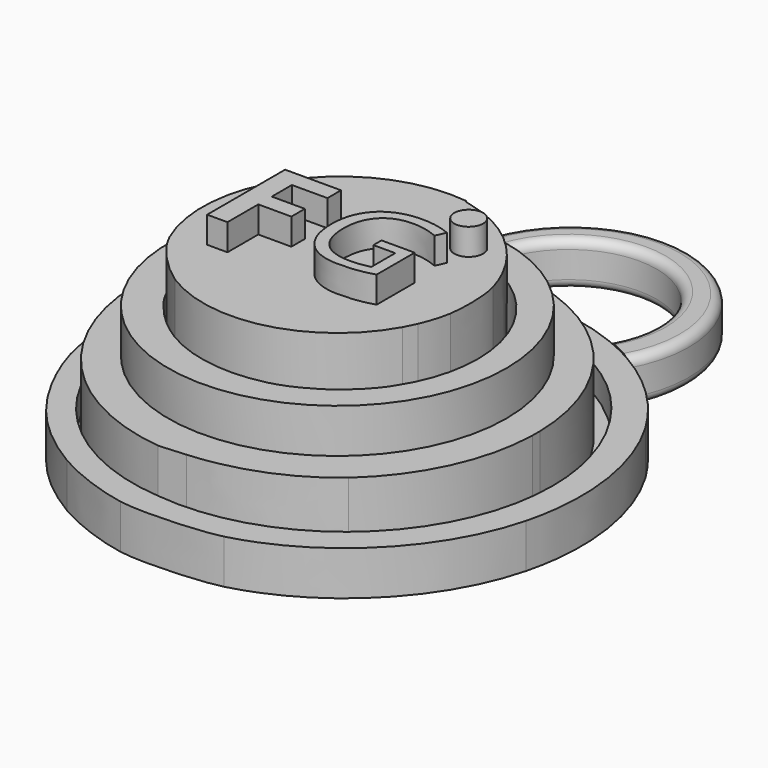
from build123d import *

# Parameters (mm, degrees)
F1_DEPTH     = 20
F0_R         = 19.1279803991
F2_DEPTH     = 15
F3_DEPTH     = 10
F4_DEPTH     = 5
F5_DEPTH     = 5
F6_R         = 1.637802748
F6_TEXT_SIZE = 15.4476677481
F7_DEPTH     = 3
F8_R         = 25.6523292118
F9_DEPTH     = 2
F10_R        = 1


# Not quite as in the source:
# - ends of sketch curves that miss each other by under 0.0002 mm in the source are joined
# - Text() gives the source's letters only with a copy of the font that has no kerning and outlines rounded to 1/6400 em; it was checked with that copy


with BuildPart() as f1:
    # F0 (on Top) → F1 (new body)
    with BuildSketch(Plane.XY):
        with BuildLine():
            ThreePointArc((-59.2347954449, -6.6814816572), (-58.8341384592, -7.4289203643), (-58.392389, -8.152832))
            add(Edge.make_bspline(
                [(-53.744252573, -12.7362436448), (-55.4325929195, -11.5891561276), (-56.9948624064, -10.0566206788), (-58.392389, -8.152832)],
                knots=[0.6895887738, 0.6895887738, 0.6895887738, 0.6895887738, 1, 1, 1, 1], degree=3))
            ThreePointArc((-53.744252573, -12.7362436448), (-41.8918676364, -14.5976951318), (-32.3863979152, -7.277170854))
            add(Edge.make_bspline(
                [(-31.7292377779, -5.9498852292), (-31.9282672637, -6.3926584279), (-32.1497491558, -6.8396976677), (-32.3863979152, -7.277170854)],
                knots=[0.3344487947, 0.3344487947, 0.3344487947, 0.3344487947, 0.5301452615, 0.5301452615, 0.5301452615, 0.5301452615], degree=3))
            ThreePointArc((-31.7292377779, -5.9498852292), (-31.1257115517, -4.3145190756), (-30.7135409768, -2.6207712256))
            add(Edge.make_bspline(
                [(-30.960104, 3.756096), (-30.5099847308, 2.24037654), (-30.4258381475, -0.5496711887), (-30.7135409768, -2.6207712256)],
                knots=[0, 0, 0, 0, 0.8296456494, 0.8296456494, 0.8296456494, 0.8296456494], degree=3))
            add(Edge.make_bspline(
                [(-42.081192, 14.696398), (-36.917409, 13.446373), (-32.566826, 9.166513), (-30.960104, 3.756096)],
                knots=[0, 0, 0, 0, 1, 1, 1, 1], degree=3))
            add(Edge.make_bspline(
                [(-43.101174, 15.090313), (-43.392217, 15.079888), (-42.933225, 14.902656), (-42.081192, 14.696398)],
                knots=[0, 0, 0, 0, 1, 1, 1, 1], degree=3))
            ThreePointArc((-43.101174, 15.090313), (-57.4988268935, 8.8957795494), (-59.2347954449, -6.6814816572))
        make_face()
    extrude(amount=F1_DEPTH)

    # F6 (on face) → F7 (join)
    with BuildSketch(Plane.XY.offset(20)):
        with Locations((-37.2399128973, 8.1431278959)):
            Circle(F6_R)
        with Locations((-57.1012012661, -5.7597728446)):
            Text('F', F6_TEXT_SIZE, font='Open Sans', font_style=FontStyle.BOLD, text_align=(TextAlign.LEFT, TextAlign.BOTTOM))
        with Locations((-46.9719469547, -5.7597728446)):
            Text('G', F6_TEXT_SIZE, font='Open Sans', text_align=(TextAlign.LEFT, TextAlign.BOTTOM))
    extrude(amount=F7_DEPTH)


with BuildPart() as f2:
    # F0 (on Top) → F2 (new body)
    with BuildSketch(Plane.XY):
        with Locations((-45.431247359, -0.1970263361)):
            Circle(F0_R)
        with BuildLine():
            add(Edge.make_bspline(
                [(-41.147337, -15.539034), (-40.1428314806, -15.2993293025), (-39.1027725479, -14.8952129249), (-38.0875846116, -14.3702912296)],
                knots=[0, 0, 0, 0, 0.285965646, 0.285965646, 0.285965646, 0.285965646], degree=3))
            add(Edge.make_bspline(
                [(-52.986997, -13.79839), (-49.483332, -15.87997), (-45.209277, -16.508342), (-41.147337, -15.539034)],
                knots=[0, 0, 0, 0, 1, 1, 1, 1], degree=3))
            add(Edge.make_bspline(
                [(-54.0793245154, -13.0384975043), (-53.6924434387, -13.339610116), (-53.3216500313, -13.5995661142), (-52.986997, -13.79839)],
                knots=[0.8132111093, 0.8132111093, 0.8132111093, 0.8132111093, 1, 1, 1, 1], degree=3))
            ThreePointArc((-54.0793245154, -13.0384975043), (-55.735609132, -11.6635433803), (-57.1866886767, -10.073529))
            add(Edge.make_bspline(
                [(-58.392389, -8.413794), (-58.1519740861, -8.8735062913), (-57.7207609953, -9.4559514121), (-57.1866886767, -10.073529)],
                knots=[0, 0, 0, 0, 0.3057410823, 0.3057410823, 0.3057410823, 0.3057410823], degree=3))
            add(Edge.make_bspline(
                [(-58.730261245, -7.7186027323), (-58.7590058786, -7.7096582658), (-58.6463817969, -7.9281163541), (-58.392389, -8.413794)],
                knots=[0.4434144709, 0.4434144709, 0.4434144709, 0.4434144709, 1, 1, 1, 1], degree=3))
            ThreePointArc((-58.730261245, -7.7186027323), (-58.9921231301, -7.2047098246), (-59.2347954449, -6.6814816572))
            ThreePointArc((-59.2347954449, -6.6814816572), (-57.8562618863, 9.1606507259), (-43.101174, 15.090313))
            add(Edge.make_bspline(
                [(-41.2900061196, 14.7616276316), (-42.0586788101, 14.9772767935), (-42.7191122675, 15.1039614431), (-43.101174, 15.090313)],
                knots=[0.5637105418, 0.5637105418, 0.5637105418, 0.5637105418, 1, 1, 1, 1], degree=3))
            ThreePointArc((-41.2900061196, 14.7616276316), (-32.7178835258, 9.2472094074), (-29.3856387082, -0.3853519649))
            ThreePointArc((-29.3856387082, -0.3853519649), (-30.0245415783, -4.8024790433), (-31.888879, -8.857532))
            add(Edge.make_bspline(
                [(-33.6493462178, -11.097555272), (-32.9505648152, -10.3812991178), (-32.3492889696, -9.624194109), (-31.888879, -8.857532)],
                knots=[0.7439800073, 0.7439800073, 0.7439800073, 0.7439800073, 1, 1, 1, 1], degree=3))
            ThreePointArc((-33.6493462178, -11.097555272), (-35.7226006868, -12.9317340256), (-38.0875846116, -14.3702912296))
        make_face(mode=Mode.SUBTRACT)
    extrude(amount=F2_DEPTH)

    # F0 (on Top) → F3 (join)
    with BuildSketch(Plane.XY):
        with BuildLine():
            Line((-47.069925, -23.475932), (-44.027216, -23.25211))
            add(Edge.make_bspline(
                [(-30.1205396487, -17.7460547966), (-33.8374032042, -20.9263141883), (-38.6163066312, -22.8540931532), (-44.027216, -23.25211)],
                knots=[0.3732264922, 0.3732264922, 0.3732264922, 0.3732264922, 1, 1, 1, 1], degree=3))
            ThreePointArc((-30.1205396487, -17.7460547966), (-24.6034613901, -10.3216274381), (-22.479647618, -1.3188673516))
            add(Edge.make_bspline(
                [(-22.475115, -0.230342), (-22.4741181138, -0.6104670398), (-22.4754785569, -0.9725951682), (-22.479647618, -1.3188673516)],
                knots=[0, 0, 0, 0, 0.0758203688, 0.0758203688, 0.0758203688, 0.0758203688], degree=3))
            ThreePointArc((-22.475115, -0.230342), (-34.5455591496, 19.4779960315), (-57.639349598, 18.5885846227))
            add(Edge.make_bspline(
                [(-63.906497, 12.228838), (-62.4986856864, 14.3385524124), (-59.8791359743, 16.9840424416), (-57.639349598, 18.5885846227)],
                knots=[0, 0, 0, 0, 0.9296926806, 0.9296926806, 0.9296926806, 0.9296926806], degree=3))
            add(Edge.make_bspline(
                [(-65.056999, 10.88216), (-65.696203, 9.619423), (-65.474943, 9.878406), (-63.906497, 12.228838)],
                knots=[0, 0, 0, 0, 1, 1, 1, 1], degree=3))
            ThreePointArc((-65.056999, 10.88216), (-65.4973944672, 10.0234562282), (-65.9020070893, 9.1473232695))
            add(Edge.make_bspline(
                [(-65.731153, 9.162373), (-65.731153, 9.2769531771), (-65.8027128579, 9.2644038713), (-65.9020070893, 9.1473232695)],
                knots=[0, 0, 0, 0, 0.7874114494, 0.7874114494, 0.7874114494, 0.7874114494], degree=3))
            add(Edge.make_bspline(
                [(-65.987633, 8.500911), (-65.846569, 8.719191), (-65.731153, 9.016851), (-65.731153, 9.162373)],
                knots=[0, 0, 0, 0, 1, 1, 1, 1], degree=3))
            add(Edge.make_bspline(
                [(-66.2406641823, 8.3307092691), (-66.2205050198, 8.2367620574), (-66.1144310132, 8.3047064339), (-65.987633, 8.500911)],
                knots=[0.10113768, 0.10113768, 0.10113768, 0.10113768, 1, 1, 1, 1], degree=3))
            ThreePointArc((-66.2406641823, 8.3307092691), (-64.5014500877, -12.3017054982), (-47.069925, -23.475932))
        make_face()
        with Locations((-45.431247359, -0.1970263361)):
            Circle(F0_R, mode=Mode.SUBTRACT)
    extrude(amount=F3_DEPTH)


with BuildPart() as f4:
    # F0 (on Top) → F4 (new body)
    with BuildSketch(Plane.XY):
        with BuildLine():
            add(Edge.make_bspline(
                [(-48.970073, -26.413517), (-51.625486, -25.940057), (-55.306082, -24.572912), (-57.588797, -23.212105)],
                knots=[0, 0, 0, 0, 1, 1, 1, 1], degree=3))
            add(Edge.make_bspline(
                [(-37.677216, -25.917347), (-40.204587, -26.574122), (-46.514432, -26.851352), (-48.970073, -26.413517)],
                knots=[0, 0, 0, 0, 1, 1, 1, 1], degree=3))
            add(Edge.make_bspline(
                [(-18.723931, -6.903355), (-21.072064, -16.0174), (-28.585257, -23.554652), (-37.677216, -25.917347)],
                knots=[0, 0, 0, 0, 1, 1, 1, 1], degree=3))
            add(Edge.make_bspline(
                [(-21.637296, 13.639865), (-17.980309, 7.51172), (-16.925794, 0.075943), (-18.723931, -6.903355)],
                knots=[0, 0, 0, 0, 1, 1, 1, 1], degree=3))
            ThreePointArc((-21.637296, 13.639865), (-25.8109452117, 18.893261801), (-31.164960657, 22.9370279049))
            ThreePointArc((-31.164960657, 22.9370279049), (-32.8667693195, 23.8327160783), (-34.6287693504, 24.6032781578))
            ThreePointArc((-34.6287693504, 24.6032781578), (-43.3302550234, 26.4435054284), (-52.1524980847, 25.3164221611))
            ThreePointArc((-52.1524980847, 25.3164221611), (-59.7026840443, 21.640329328), (-65.733156707, 15.7963267608))
            add(Edge.make_bspline(
                [(-69.2860531049, 9.3594504448), (-68.3414214755, 11.7099431853), (-67.1463052527, 13.8651148137), (-65.733156707, 15.7963267608)],
                knots=[0.0254254095, 0.0254254095, 0.0254254095, 0.0254254095, 0.2859602016, 0.2859602016, 0.2859602016, 0.2859602016], degree=3))
            ThreePointArc((-69.2860531049, 9.3594504448), (-69.4192204262, 9.0043367676), (-69.547318, 8.647363))
            ThreePointArc((-69.547318, 8.647363), (-70.144466641, 6.7128124545), (-70.5929494637, 4.7384934654))
            add(Edge.make_bspline(
                [(-69.40493, -9.153827), (-71.00351631, -5.1220863609), (-71.4043965437, 0.1179787787), (-70.5929494637, 4.7384934654)],
                knots=[0, 0, 0, 0, 0.7708246728, 0.7708246728, 0.7708246728, 0.7708246728], degree=3))
            add(Edge.make_bspline(
                [(-57.588797, -23.212105), (-63.292625, -19.811874), (-66.863546, -15.563365), (-69.40493, -9.153827)],
                knots=[0, 0, 0, 0, 1, 1, 1, 1], degree=3))
        make_face()
        with BuildLine():
            ThreePointArc((-21.0622935478, -0.2228973471), (-28.8652464336, -17.66638119), (-47.069925, -23.475932))
            ThreePointArc((-47.069925, -23.475932), (-65.5880574373, -11.2831815996), (-65.056999, 10.88216))
            add(Edge.make_bspline(
                [(-53.02305, 21.71414), (-57.817765, 19.865098), (-62.763129, 15.413691), (-65.056999, 10.88216)],
                knots=[0, 0, 0, 0, 1, 1, 1, 1], degree=3))
            add(Edge.make_bspline(
                [(-34.119623, 20.950198), (-39.888503, 23.76455), (-46.964626, 24.050518), (-53.02305, 21.71414)],
                knots=[0, 0, 0, 0, 1, 1, 1, 1], degree=3))
            add(Edge.make_bspline(
                [(-21.879548, 5.907178), (-23.680713, 12.54305), (-28.152859, 18.039306), (-34.119623, 20.950198)],
                knots=[0, 0, 0, 0, 1, 1, 1, 1], degree=3))
            ThreePointArc((-21.879548, 5.907178), (-21.2675070442, 2.8692592062), (-21.0622935478, -0.2228973471))
        make_face(mode=Mode.SUBTRACT)
    extrude(amount=F4_DEPTH)


with BuildPart() as f5:
    # F0 (on Top) → F5 (new body)
    with BuildSketch(Plane.XY):
        with BuildLine():
            add(Edge.make_bspline(
                [(-34.5666196684, 24.7092430798), (-33.3810366932, 24.2207005987), (-32.2320034389, 23.6484291155), (-31.1295313761, 23.0001864934)],
                knots=[0.1322045887, 0.1322045887, 0.1322045887, 0.1322045887, 0.3238140526, 0.3238140526, 0.3238140526, 0.3238140526], degree=3))
            ThreePointArc((-31.1295313761, 23.0001864934), (-42.0731684167, 42.8839416727), (-55.1710537864, 24.3482380025))
            add(Edge.make_bspline(
                [(-55.1710537864, 24.3482380025), (-54.2149744978, 24.769792958), (-53.2281255532, 25.1355815735), (-52.2133910902, 25.4430586472)],
                knots=[0.7959745665, 0.7959745665, 0.7959745665, 0.7959745665, 0.9122414491, 0.9122414491, 0.9122414491, 0.9122414491], degree=3))
            ThreePointArc((-52.2133910902, 25.4430586472), (-42.7834765104, 39.6619361545), (-34.5666196684, 24.7092430798))
        make_face()
    extrude(amount=F5_DEPTH)

    # F10
    f10_edges = [f5.edges().sort_by_distance(p)[0] for p in [
        (-42.783477, 39.661936, 0),
        (-42.783477, 39.661936, 5),
        (-42.073168, 42.883942, 5),
        (-42.073168, 42.883942, 0),
    ]]
    fillet(f10_edges, radius=F10_R)


with BuildPart() as f9:
    # F8 (on Top) → F9 (new body)
    with BuildSketch(Plane.XY):
        with Locations((-44.544095667, -0.2898088063)):
            Circle(F8_R)
    extrude(amount=F9_DEPTH)


solid = Compound([f1.part, f2.part, f4.part, f5.part, f9.part])
